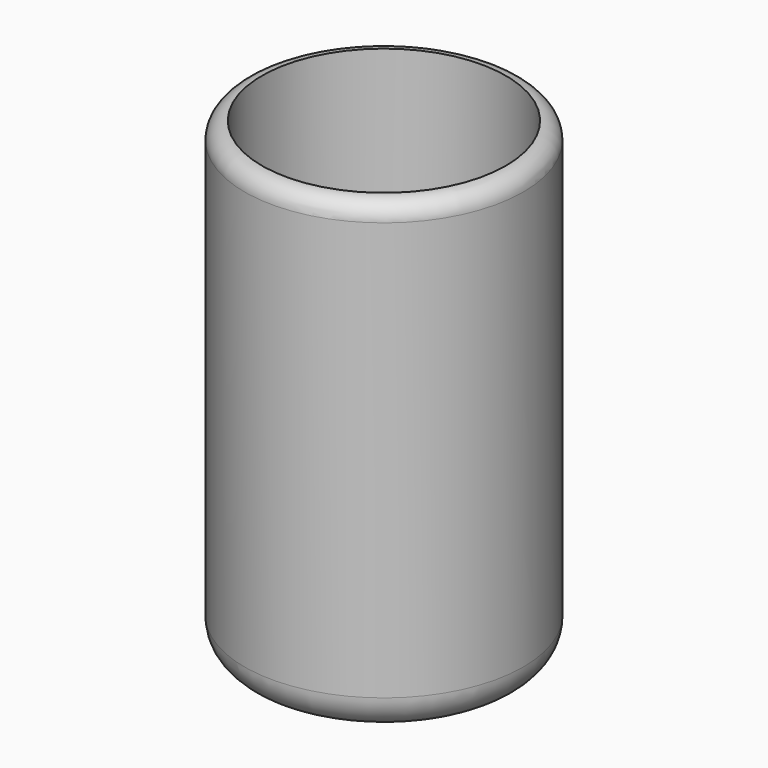
from build123d import *

# Parameters (mm, degrees)
F0_W   = 35
F0_H   = 10
F0_W_2 = 5
F0_H_2 = 125
F2_R   = 4.99999
F3_R   = 10


# Not quite as in the source:
# - a fillet or chamfer is up to 0.001 mm smaller than in the source, because OpenCascade refuses the exact size


with BuildPart() as f1:
    # F0 (on Front) → F1 (revolve)
    with BuildSketch(Plane.XZ):
        with Locations((17.5, 5)):
            Rectangle(F0_W, F0_H)
        with Locations((37.5, 5)):
            Rectangle(F0_W_2, F0_H)
        with Locations((37.5, 72.5)):
            Rectangle(F0_W_2, F0_H_2)
    revolve(axis=Axis((0, 0, 5), (0, 0, -1)))

    # F2 (radius 5 in the source; OpenCascade refuses exactly that, so slightly less here)
    f2_edges = [f1.edges().sort_by_distance(p)[0] for p in [
        (-40, 0, 135),
    ]]
    fillet(f2_edges, radius=F2_R)

    # F3
    f3_edges = [f1.edges().sort_by_distance(p)[0] for p in [
        (-40, 0, 0),
    ]]
    fillet(f3_edges, radius=F3_R)


solid = f1.part
